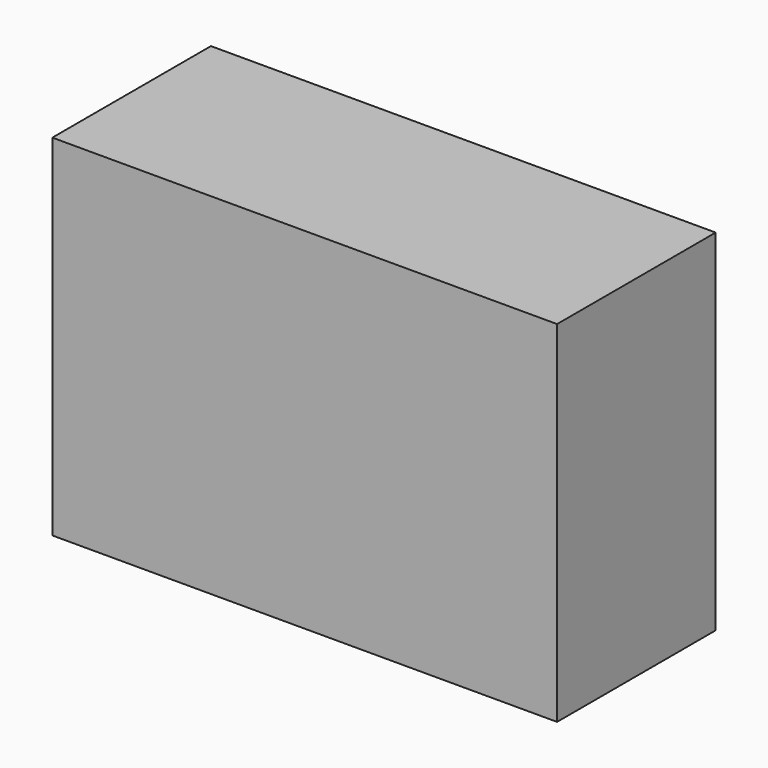
from build123d import *

# Parameters (mm, degrees)
F0_W     = 64.6750666201
F0_H     = 44.87657547
F1_DEPTH = 25.4


# Not quite as in the source:
# - the program builds the solid bodies; features that only make, move or delete a surface that nothing else refers to are left out


with BuildPart() as f1:
    # F0 (on Front) → F1 (new body)
    with BuildSketch(Plane.XZ):
        with Locations((-81.7017685622, 49.4962260127)):
            Rectangle(F0_W, F0_H)
    extrude(amount=F1_DEPTH)


solid = f1.part
